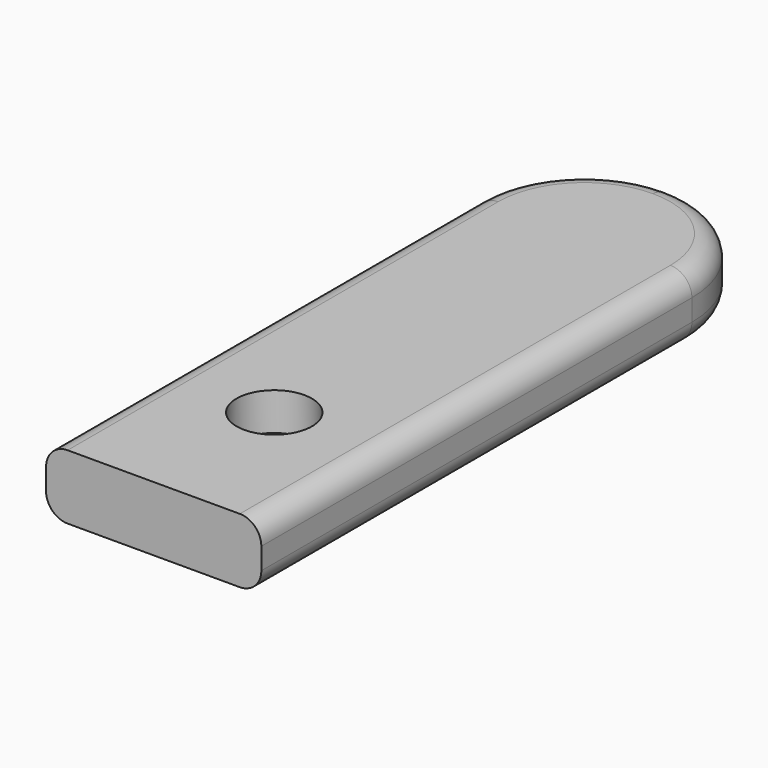
from build123d import *

# Parameters (mm, degrees)
F0_W           = 10
F0_H           = 30
F1_DEPTH       = 3
F2_D           = 3.5
F2_DEPTH       = 3
F2_CSINK_D     = 6
F2_CSINK_ANGLE = 90
F2_TIP         = 1.0515060833
F3_R           = 4.99999
F4_R           = 1


# Not quite as in the source:
# - a fillet or chamfer is up to 0.001 mm smaller than in the source, because OpenCascade refuses the exact size


with BuildPart() as f1:
    # F0 (on Top) → F1 (new body)
    with BuildSketch(Plane.XY):
        with Locations((0, 15)):
            Rectangle(F0_W, F0_H)
    extrude(amount=F1_DEPTH)

    # F2
    with Locations(Plane(origin=(0, 0, 0), x_dir=(1, 0, 0), z_dir=(0, 0, -1))):
        with Locations((0, -7)):
            CounterSinkHole(F2_D / 2, F2_CSINK_D / 2, depth=F2_DEPTH, counter_sink_angle=F2_CSINK_ANGLE)
            with Locations((0, 0, -(F2_DEPTH + F2_TIP / 2))):  # 118° drill point
                Cone(0, F2_D / 2, F2_TIP, mode=Mode.SUBTRACT)

    # F3 (radius 5 in the source; OpenCascade refuses exactly that, so slightly less here)
    f3_edges = [f1.edges().sort_by_distance(p)[0] for p in [
        (5, 30, 1.5),
        (-5, 30, 1.5),
    ]]
    fillet(f3_edges, radius=F3_R)

    # F4
    f4_edges = [f1.edges().sort_by_distance(p)[0] for p in [
        (3.535537, 28.535537, 0),
        (3.535537, 28.535537, 3),
        (-5, 12.500005, 3),
        (5, 12.500005, 3),
    ]]
    fillet(f4_edges, radius=F4_R)


solid = f1.part
